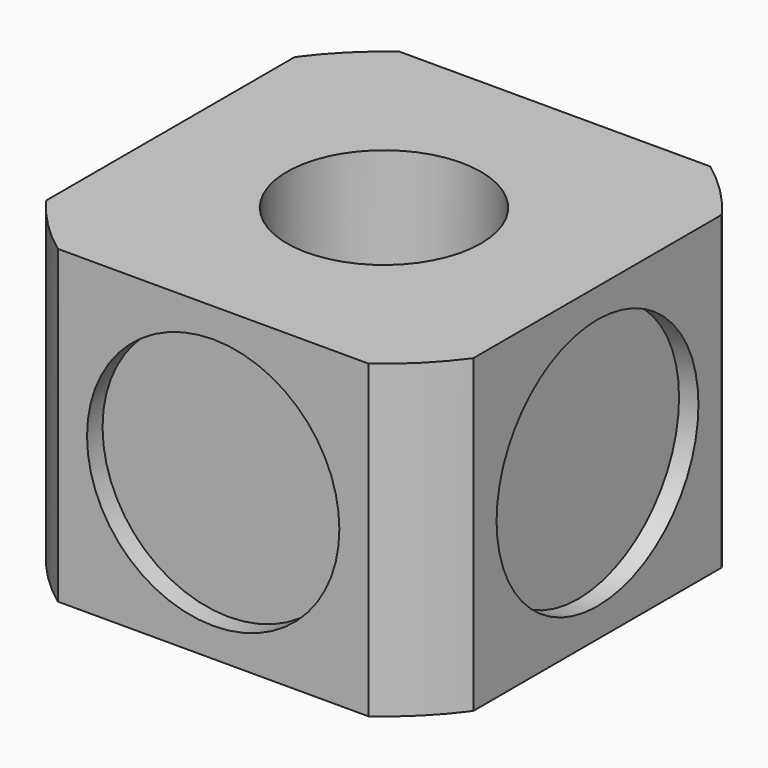
from build123d import *

# Parameters (mm, degrees)
F0_R            = 5
F2_DEPTH        = 16
F3_R            = 6.5
F4_DEPTH        = 1
F4_COPIES_COUNT = 4
F0_R_2          = 2.5
F5_DEPTH        = 3


# Not quite as in the source:
# - a pattern or mirror of a feature is missing from the dataset's text; its kind, count and spacing are read off the source's solid


with BuildPart() as f2:
    # F0 (on Top) → F2 (new body)
    with BuildSketch(Plane.XY):
        with BuildLine():
            Line((11, -8), (11, 8))
            ThreePointArc((11, 8), (9.6176920308, 9.6176920308), (8, 11))
            Line((8, 11), (-8, 11))
            ThreePointArc((-8, 11), (-9.6176920308, 9.6176920308), (-11, 8))
            Line((-11, 8), (-11, -8))
            ThreePointArc((-11, -8), (-9.6176920308, -9.6176920308), (-8, -11))
            Line((-8, -11), (8, -11))
            ThreePointArc((8, -11), (9.6176920308, -9.6176920308), (11, -8))
        make_face()
        Circle(F0_R, mode=Mode.SUBTRACT)
    extrude(amount=F2_DEPTH)

    # F3 (on face) → F4 (cut)
    with BuildSketch(Plane.XZ.offset(11)):
        with Locations((0, 8)):
            Circle(F3_R)
    f4 = extrude(amount=-F4_DEPTH, mode=Mode.SUBTRACT)

    # F4_copies: F4 ×4 about axis
    f4_copies_axis = Axis((0, 0, 0), (0, 0, 1))
    for i in range(1, F4_COPIES_COUNT):
        add(f4.rotate(f4_copies_axis, i * 360 / F4_COPIES_COUNT), mode=Mode.SUBTRACT)

    # F0 (on Top) → F5 (join)
    with BuildSketch(Plane.XY):
        Circle(F0_R)
        Circle(F0_R_2, mode=Mode.SUBTRACT)
    extrude(amount=F5_DEPTH)


solid = f2.part
